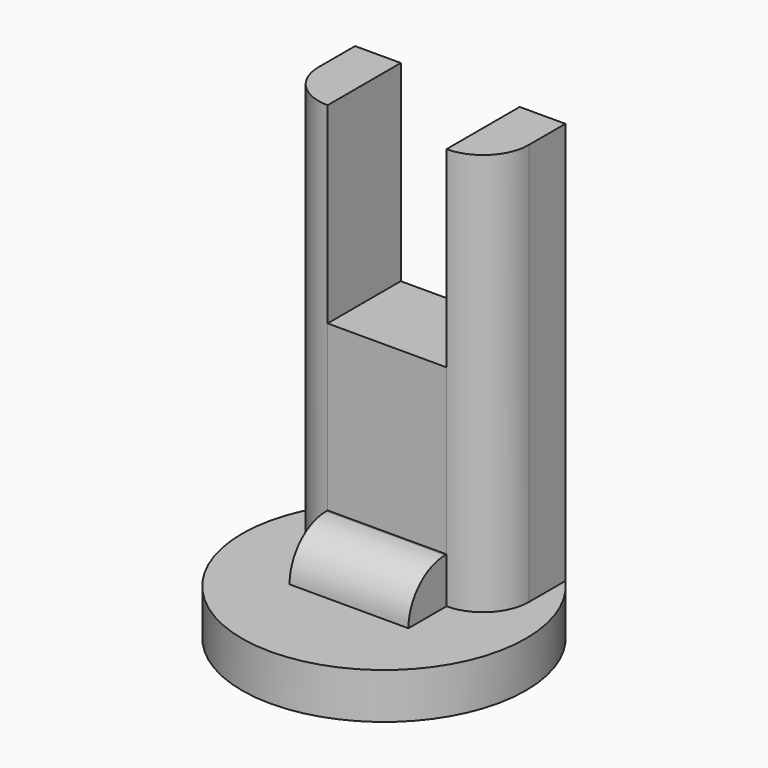
from build123d import *

# Parameters (mm, degrees)
F1_DEPTH = 10
F3_DEPTH = 5
F4_R     = 5
F5_W     = 13
F5_H     = 5.2037292719
F6_DEPTH = 5
F7_R     = 4.99999


# Not quite as in the source:
# - a fillet or chamfer is up to 0.001 mm smaller than in the source, because OpenCascade refuses the exact size


with BuildPart() as f1:
    # F0 (on Front) → F1 (new body)
    with BuildSketch(Plane.XZ):
        Polygon((-10.9377613165, 42.7635207549), (-15.9377613165, 42.7635207549), (-15.9377613165, -6.2364792451), (7.0622386835, -6.2364792451), (7.0622386835, 42.7635207549), (2.0622386835, 42.7635207549), (2.0622386835, 21.7635207549), (-10.9377613165, 21.7635207549), align=None)
    extrude(amount=F1_DEPTH)

    # F2 (on face) → F3 (join)
    with BuildSketch(Plane(origin=(0, 0, -6.2364792451), x_dir=(1, 0, 0), z_dir=(0, 0, -1))):
        with BuildLine():
            Line((7.0622386835, 10), (7.0622386835, 0))
            ThreePointArc((7.0622386835, 0), (-4.4377613165, 25.9396283258), (-15.9377613165, 0))
            Line((-15.9377613165, 0), (-15.9377613165, 10))
            Line((-15.9377613165, 10), (7.0622386835, 10))
        make_face()
    extrude(amount=-F3_DEPTH)

    # F4
    f4_edges = [f1.edges().sort_by_distance(p)[0] for p in [
        (-15.937761, -10, 20.763521),
        (7.062239, -10, 20.763521),
    ]]
    fillet(f4_edges, radius=F4_R)

    # F5 (on face) → F6 (join)
    with BuildSketch(Plane.XY.offset(-1.2364792451)):
        with Locations((-4.4377613165, -12.6018646359)):
            Rectangle(F5_W, F5_H)
    extrude(amount=F6_DEPTH)

    # F7 (radius 5 in the source; OpenCascade refuses exactly that, so slightly less here)
    f7_edges = [f1.edges().sort_by_distance(p)[0] for p in [
        (-4.437761, -15.203729, 3.763521),
    ]]
    fillet(f7_edges, radius=F7_R)


solid = f1.part
